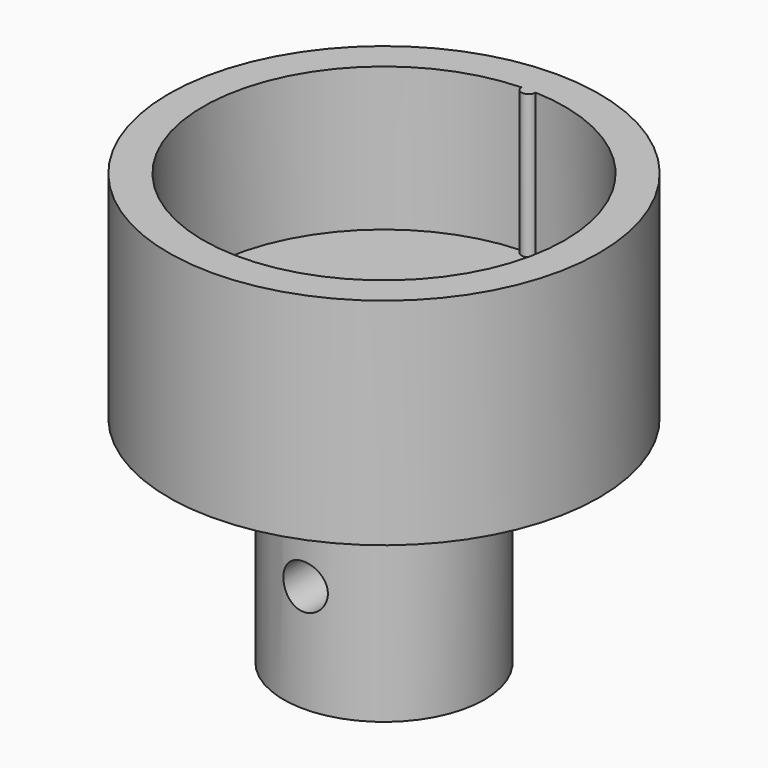
from build123d import *

# Parameters (mm, degrees)
F0_R     = 7
F1_DEPTH = 15
F2_DEPTH = 5
F0_R_2   = 15
F3_DEPTH = 15
F5_D     = 3.1
F5_DEPTH = 13.201
F6_DEPTH = 15
F7_W     = 7
F7_H     = 7
F8_DEPTH = 3


with BuildPart() as f1:
    # F0 (on Top) → F1 (new body)
    with BuildSketch(Plane.XY):
        Circle(F0_R)
        with BuildLine():
            Line((2.0124611797, -1.8), (-2.0124611797, -1.8))
            ThreePointArc((-2.0124611797, -1.8), (0, 2.7), (2.0124611797, -1.8))
        make_face(mode=Mode.SUBTRACT)
    extrude(amount=-F1_DEPTH)

    # F0 (on Top) → F2 (join)
    with BuildSketch(Plane.XY):
        with BuildLine():
            ThreePointArc((-0.4999015713, 12.5900793651), (-8.731014838, -9.0845682286), (12.6, 0))
            ThreePointArc((12.6, 0), (9.0845682286, 8.731014838), (0.4999015713, 12.5900793651))
            ThreePointArc((0.4999015713, 12.5900793651), (0, 12.1), (-0.4999015713, 12.5900793651))
        make_face()
        Circle(F0_R, mode=Mode.SUBTRACT)
        Circle(F0_R)
        with BuildLine():
            Line((2.0124611797, -1.8), (-2.0124611797, -1.8))
            ThreePointArc((-2.0124611797, -1.8), (0, 2.7), (2.0124611797, -1.8))
        make_face(mode=Mode.SUBTRACT)
        with BuildLine():
            ThreePointArc((2.0124611797, -1.8), (0, 2.7), (-2.0124611797, -1.8))
            Line((-2.0124611797, -1.8), (2.0124611797, -1.8))
        make_face()
    extrude(amount=F2_DEPTH)

    # F0 (on Top) → F3 (join)
    with BuildSketch(Plane.XY):
        Circle(F0_R_2)
        with BuildLine():
            ThreePointArc((0.4999015713, 12.5900793651), (9.0845682286, 8.731014838), (12.6, 0))
            ThreePointArc((12.6, 0), (-8.731014838, -9.0845682286), (-0.4999015713, 12.5900793651))
            ThreePointArc((-0.4999015713, 12.5900793651), (0, 12.6), (0.4999015713, 12.5900793651))
        make_face(mode=Mode.SUBTRACT)
    extrude(amount=F3_DEPTH)

    # F5 (through all, one way)
    with BuildSketch(Plane(origin=(0, -1.8, 0), x_dir=(-1, 0, 0), z_dir=(0, 1, 0))):
        with Locations((0, -7.5)):
            Circle(F5_D / 2)
    extrude(amount=-F5_DEPTH, mode=Mode.SUBTRACT)

    # F0 (on Top) → F6 (join)
    with BuildSketch(Plane.XY):
        with BuildLine():
            ThreePointArc((-0.4999015713, 12.5900793651), (0, 12.1), (0.4999015713, 12.5900793651))
            ThreePointArc((0.4999015713, 12.5900793651), (0, 12.6), (-0.4999015713, 12.5900793651))
        make_face()
    extrude(amount=F6_DEPTH)

    # F7 (on face) → F8 (cut)
    with BuildSketch(Plane.XY.offset(5)):
        Rectangle(F7_W, F7_H)
    extrude(amount=-F8_DEPTH, mode=Mode.SUBTRACT)


solid = f1.part
